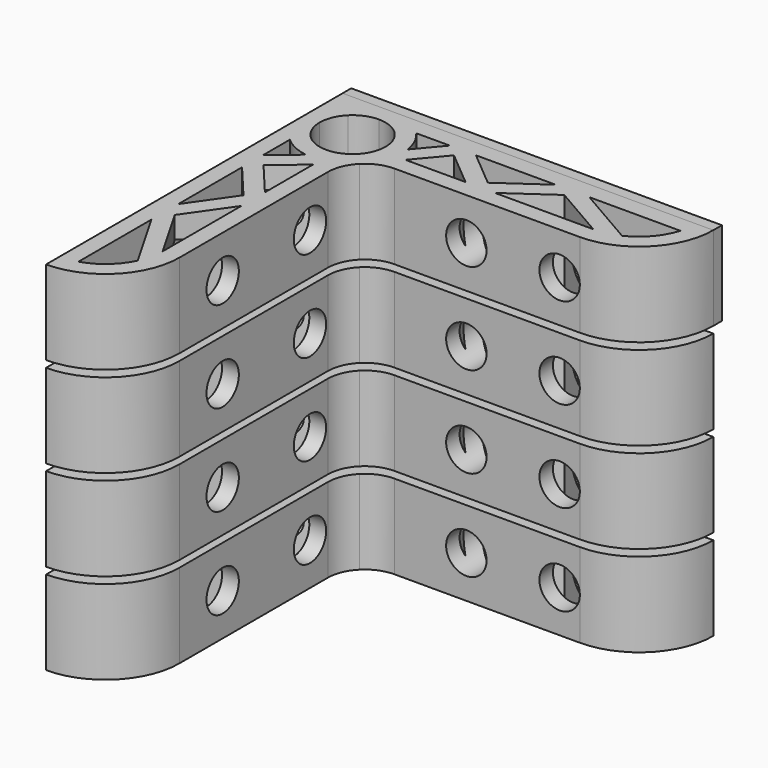
from build123d import *
from build123d import SkipClean  # not in build123d's __all__

# Parameters (mm, degrees)
F1_DEPTH  = 25
F3_R      = 3.25
F5_DEPTH  = 25
F6_START  = -7
F3_R_2    = 6
F6_DEPTH  = 18
F4_R      = 2.25
F7_DEPTH  = 25
F8_START  = -6.3
F4_R_2    = 6
F8_DEPTH  = 18.7
F9_SIZE   = 2
F13_R     = 0.6384973242
F14_DEPTH = 106
F15_DEPTH = 3.2


with BuildPart() as f1:
    # F0 (on Top) → F1 (new body)
    with BuildSketch(Plane.XY):
        with BuildLine():
            Line((7.8629150102, 102.1370849898), (5, 105))
            Line((5, 105), (5, 95.2253967444))
            ThreePointArc((5, 95.2253967444), (5.7440473693, 98.9659754683), (7.8629150102, 102.1370849898))
        make_face()
        with BuildLine():
            Line((0, 110), (0, 0))
            ThreePointArc((0, 0), (15.5563491861, 6.4436508139), (22, 22))
            Line((22, 22), (22, 77))
            ThreePointArc((22, 77), (22.8373251424, 81.209517756), (25.2218254069, 84.7781745931))
            Line((25.2218254069, 84.7781745931), (21.686291501, 88.313708499))
            ThreePointArc((21.686291501, 88.313708499), (21.463593918, 88.0865384459), (21.2454568407, 87.8549857262))
            ThreePointArc((21.2454568407, 87.8549857262), (18.2459547541, 83.1901654971), (17.019102823, 77.7816171821))
            ThreePointArc((17.019102823, 77.7816171821), (17.0047764187, 77.3909252925), (17, 77))
            Line((17, 77), (17, 59.9223857717))
            Line((17, 59.9223857717), (17, 51.2051517936))
            Line((17, 51.2051517936), (17, 22))
            ThreePointArc((17, 22), (16.5932784973, 18.3036357443), (15.3925754457, 14.7841409973))
            ThreePointArc((15.3925754457, 14.7841409973), (11.1516600986, 9.1687694649), (5, 5.7519231907))
            Line((5, 5.7519231907), (5, 32.7846096908))
            Line((5, 32.7846096908), (5, 42.7846096908))
            Line((5, 42.7846096908), (5, 66.4448097486))
            Line((5, 66.4448097486), (5, 74.2234288829))
            Line((5, 74.2234288829), (5, 84.146315891))
            Line((5, 84.146315891), (5, 95.2253967444))
            Line((5, 95.2253967444), (5, 105))
            Line((5, 105), (0, 110))
        make_face()
        with BuildLine():
            ThreePointArc((21.686291501, 88.313708499), (11.0340245317, 86.1948408582), (5, 95.2253967444))
            Line((5, 95.2253967444), (5, 84.146315891))
            ThreePointArc((5, 84.146315891), (8.5492541846, 81.8263695295), (12.6112589896, 80.6100334938))
            Line((12.6112589896, 80.6100334938), (21.2454568407, 87.8549857262))
            ThreePointArc((21.2454568407, 87.8549857262), (21.463593918, 88.0865384459), (21.686291501, 88.313708499))
        make_face()
        with BuildLine():
            ThreePointArc((17.019102823, 77.7816171821), (18.2459547541, 83.1901654971), (21.2454568407, 87.8549857262))
            Line((21.2454568407, 87.8549857262), (12.6112589896, 80.6100334938))
            Line((12.6112589896, 80.6100334938), (5, 74.2234288829))
            Line((5, 74.2234288829), (8.2139380484, 70.3932066673))
            Line((8.2139380484, 70.3932066673), (17, 77.7655880103))
            Line((17, 77.7655880103), (17.019102823, 77.7816171821))
        make_face()
        Polygon((8.2139380484, 70.3932066673), (5, 74.2234288829), (5, 66.4448097486), (14.030949889, 55.6821427738), (17, 59.9223857717), align=None)
        Polygon((14.030949889, 55.6821427738), (5, 42.7846096908), (7.7584447974, 38.0068431518), (17, 51.2051517936), (17, 59.9223857717), align=None)
        with BuildLine():
            Line((7.7584447974, 38.0068431518), (5, 42.7846096908))
            Line((5, 42.7846096908), (5, 32.7846096908))
            Line((5, 32.7846096908), (15.3925754457, 14.7841409973))
            ThreePointArc((15.3925754457, 14.7841409973), (16.5932784973, 18.3036357443), (17, 22))
            Line((17, 22), (7.7584447974, 38.0068431518))
        make_face()
    extrude(amount=F1_DEPTH)

    # F2: F1 across face


with BuildPart() as f1_1:
    add(f1.part, clean=False)
    with SkipClean():  # cleaning this boolean's faces spoils the solid; the shape is the same uncleaned
        add(f1.part.mirror(Plane(origin=(3.9314575051, 106.0685424949, 12.5), x_dir=(-0.7071067812, 0.7071067812, 0), z_dir=(0.7071067812, 0.7071067812, 0))), clean=False)

    # F3 (on face) → F5 (cut)
    with BuildSketch(Plane(origin=(0, 0, 0), x_dir=(0, -1, 0), z_dir=(-1, 0, 0))):
        with Locations((-70.3932066673, 12.5)):
            Circle(F3_R)
        with Locations((-38.0068431518, 12.5)):
            Circle(F3_R)
    extrude(amount=-F5_DEPTH, mode=Mode.SUBTRACT)

    # F3 (on face) → F6 (cut)
    with BuildSketch(Plane(origin=(0, 0, 0), x_dir=(0, -1, 0), z_dir=(-1, 0, 0)).offset(F6_START)):
        with Locations((-70.3932066673, 12.5)):
            Circle(F3_R_2)
        with Locations((-70.3932066673, 12.5)):
            Circle(F3_R, mode=Mode.SUBTRACT)
        with Locations((-38.0068431518, 12.5)):
            Circle(F3_R_2)
        with Locations((-38.0068431518, 12.5)):
            Circle(F3_R, mode=Mode.SUBTRACT)
    extrude(amount=-F6_DEPTH, mode=Mode.SUBTRACT)

    # F4 (on face) → F7 (cut)
    with BuildSketch(Plane(origin=(0, 110, 0), x_dir=(-1, 0, 0), z_dir=(0, 1, 0))):
        with Locations((-82, 12.5)):
            Circle(F4_R)
        with Locations((-54.3178572262, 12.5)):
            Circle(F4_R)
    extrude(amount=-F7_DEPTH, mode=Mode.SUBTRACT)

    # F4 (on face) → F8 (cut)
    with BuildSketch(Plane(origin=(0, 110, 0), x_dir=(-1, 0, 0), z_dir=(0, 1, 0)).offset(F8_START)):
        with Locations((-54.3178572262, 12.5)):
            Circle(F4_R_2)
        with Locations((-54.3178572262, 12.5)):
            Circle(F4_R, mode=Mode.SUBTRACT)
        with Locations((-82, 12.5)):
            Circle(F4_R_2)
        with Locations((-82, 12.5)):
            Circle(F4_R, mode=Mode.SUBTRACT)
    extrude(amount=-F8_DEPTH, mode=Mode.SUBTRACT)

    # F9
    f9_edges = [f1_1.edges().sort_by_distance(p)[0] for p in [
        (56.567857, 105, 12.5),
        (84.25, 105, 12.5),
    ]]
    chamfer(f9_edges, length=F9_SIZE)


with BuildPart() as f10_1:
    # F10: copy of F1
    add(f1_1.part.moved(Location((0, 0, 27))), clean=False)


with BuildPart() as f11_1:
    # F11: copy of F10_1
    add(f10_1.part.moved(Location((0, 0, 27))), clean=False)


with BuildPart() as f12_1:
    # F12: copy of F11_1
    add(f11_1.part.moved(Location((0, 0, 27))), clean=False)


with BuildPart() as f1_2:
    add(f1_1.part, clean=False)

    add(f10_1.part)  # F14 merges F10_1

    add(f11_1.part)  # F14 merges F11_1

    add(f12_1.part)  # F14 merges F12_1
    # F13 (on face) → F14 (join, through all)
    with BuildSketch(Plane.XY.offset(106)):
        with Locations((3.7311331835, 105.9773936868)):
            Circle(F13_R)
    extrude(amount=-F14_DEPTH)


with BuildPart() as f15:
    # F15 (new): a face of the model
    f15_faces = [f1_2.part.faces().sort_by_distance(p)[0] for p in [
        (1.1280514173, 110, 93.5),
    ]]
    extrude(f15_faces, amount=F15_DEPTH)


solid = Compound([f1_2.part, f15.part])
